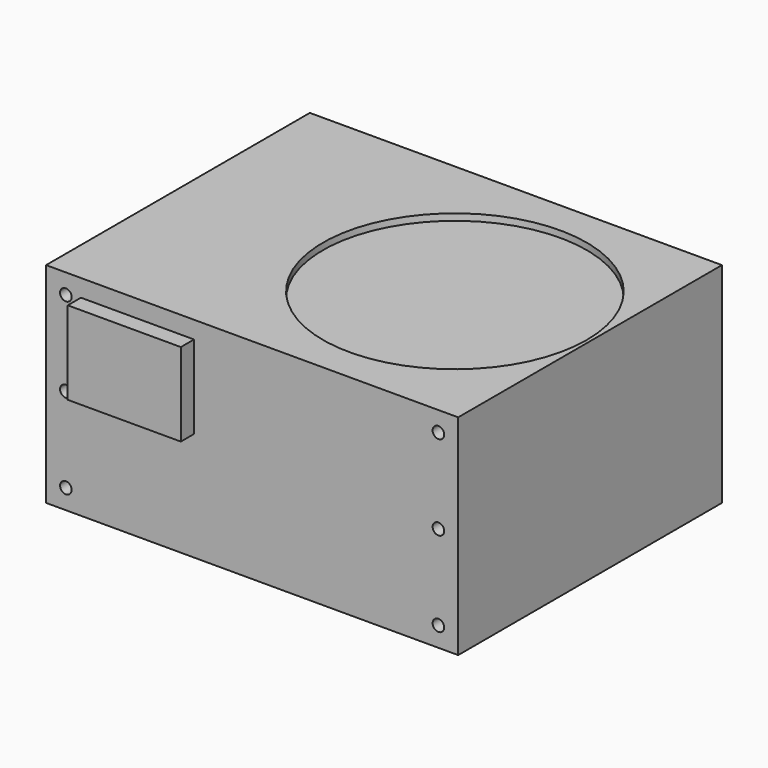
from build123d import *

# Parameters (mm, degrees)
F0_W     = 125
F0_H     = 63.5
F0_R     = 1.755
F0_W_2   = 34.3037378043
F0_H_2   = 25.238768314
F1_DEPTH = 100
F2_DEPTH = 5
F3_DEPTH = 5
F4_R     = 40
F5_DEPTH = 2


# Not quite as in the source:
# - a feature names something its author has since deleted; it is built from what else it names


with BuildPart() as f1:
    # F0 (on Front) → F1 (new body)
    with BuildSketch(Plane.XZ):
        Rectangle(F0_W, F0_H)
        with Locations((-56.5, -25.75)):
            Circle(F0_R, mode=Mode.SUBTRACT)
        with Locations((56.5, -25.75)):
            Circle(F0_R, mode=Mode.SUBTRACT)
        with Locations((-56.5, 0)):
            Circle(F0_R, mode=Mode.SUBTRACT)
        with Locations((-34.777761437, 13.8649413711)):
            Rectangle(F0_W_2, F0_H_2, mode=Mode.SUBTRACT)
        with Locations((-56.5, 25.75)):
            Circle(F0_R, mode=Mode.SUBTRACT)
        with Locations((56.5, 0)):
            Circle(F0_R, mode=Mode.SUBTRACT)
        with Locations((56.5, 25.75)):
            Circle(F0_R, mode=Mode.SUBTRACT)
        with Locations((-34.777761437, 13.8649413711)):
            Rectangle(F0_W_2, F0_H_2)
        with Locations((-56.5, 25.75)):
            Circle(F0_R)
        with Locations((-56.5, 0)):
            Circle(F0_R)
        with Locations((-56.5, -25.75)):
            Circle(F0_R)
        with Locations((56.5, -25.75)):
            Circle(F0_R)
        with Locations((56.5, 0)):
            Circle(F0_R)
        with Locations((56.5, 25.75)):
            Circle(F0_R)
    extrude(amount=-F1_DEPTH)

    # F0 (on Front) → F2 (join)
    with BuildSketch(Plane.XZ):
        with Locations((-34.777761437, 13.8649413711)):
            Rectangle(F0_W_2, F0_H_2)
    extrude(amount=F2_DEPTH)

    # F0 (on Front) → F3 (cut)
    with BuildSketch(Plane.XZ):
        with Locations((-56.5, 25.75)):
            Circle(F0_R)
        with Locations((-56.5, 0)):
            Circle(F0_R)
        with Locations((-56.5, -25.75)):
            Circle(F0_R)
        with Locations((56.5, -25.75)):
            Circle(F0_R)
        with Locations((56.5, 0)):
            Circle(F0_R)
        with Locations((56.5, 25.75)):
            Circle(F0_R)
    extrude(amount=-F3_DEPTH, mode=Mode.SUBTRACT)

    # F4 (on face) → F5 (cut)
    with BuildSketch(Plane.XY.offset(31.75)):
        with Locations((21.5, 50)):
            Circle(F4_R)
    extrude(amount=-F5_DEPTH, mode=Mode.SUBTRACT)


solid = f1.part
